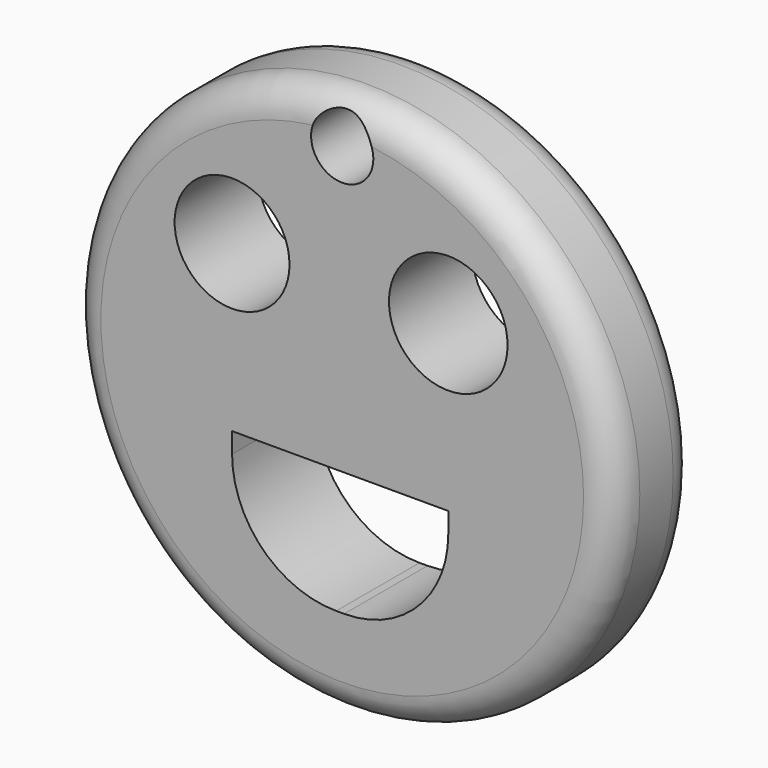
from build123d import *

# Parameters (mm, degrees)
F0_R     = 26.177757608
F0_R_2   = 5.5155489558
F0_R_3   = 2.9897173108
F0_R_4   = 5.6935154322
F1_DEPTH = 10


# Not quite as in the source:
# - a fillet or chamfer that OpenCascade refuses, or shapes differently, is made with other operations: its cross-section is extruded or revolved along the edge and cut away or added


with BuildPart() as f1:
    # F0 (on Front) → F1 (new body)
    with BuildSketch(Plane.XZ):
        Circle(F0_R)
        with BuildLine():
            Line((-10.5765974149, -7.333868891), (-10.5765974149, -5.3862300701))
            Line((-10.5765974149, -5.3862300701), (10.1848710328, -5.3862300701))
            Line((10.1848710328, -5.3862300701), (10.1848710328, -7.333868891))
            ThreePointArc((10.1848710328, -7.333868891), (7.2559388447, -14.4049367029), (0.1848710328, -17.333868891))
            Line((0.1848710328, -17.333868891), (-0.5765974149, -17.333868891))
            ThreePointArc((-0.5765974149, -17.333868891), (-7.6476652268, -14.4049367029), (-10.5765974149, -7.333868891))
        make_face(mode=Mode.SUBTRACT)
        with Locations((-10.5765974149, 10.4786651209)):
            Circle(F0_R_2, mode=Mode.SUBTRACT)
        with Locations((0, 22.0345780253)):
            Circle(F0_R_3, mode=Mode.SUBTRACT)
        with Locations((10.1848710328, 10.4786651209)):
            Circle(F0_R_4, mode=Mode.SUBTRACT)
    extrude(amount=F1_DEPTH)

    # F2: fillet of radius 3 on 2 edges, made by hand

    # F2_s1 → F2_t2 (revolve, cut)
    with BuildSketch(Plane.XY):
        with BuildLine():
            ThreePointArc((26.177757608, -7), (25.2990779516, -9.1213203436), (23.177757608, -10))
            Line((23.177757608, -10), (26.177757608, -10))
            Line((26.177757608, -10), (26.177757608, -7))
        make_face()
    revolve(axis=Axis((0, -10, 0), (0, -1, 0)), mode=Mode.SUBTRACT)

    # F2_s3 → F2_t4 (revolve, cut)
    with BuildSketch(Plane.XY):
        with BuildLine():
            ThreePointArc((26.177757608, -3), (25.2990779516, -0.8786796564), (23.177757608, 0))
            Line((23.177757608, 0), (26.177757608, 0))
            Line((26.177757608, 0), (26.177757608, -3))
        make_face()
    revolve(axis=Axis((0, 0, 0), (0, -1, 0)), mode=Mode.SUBTRACT)


solid = f1.part
